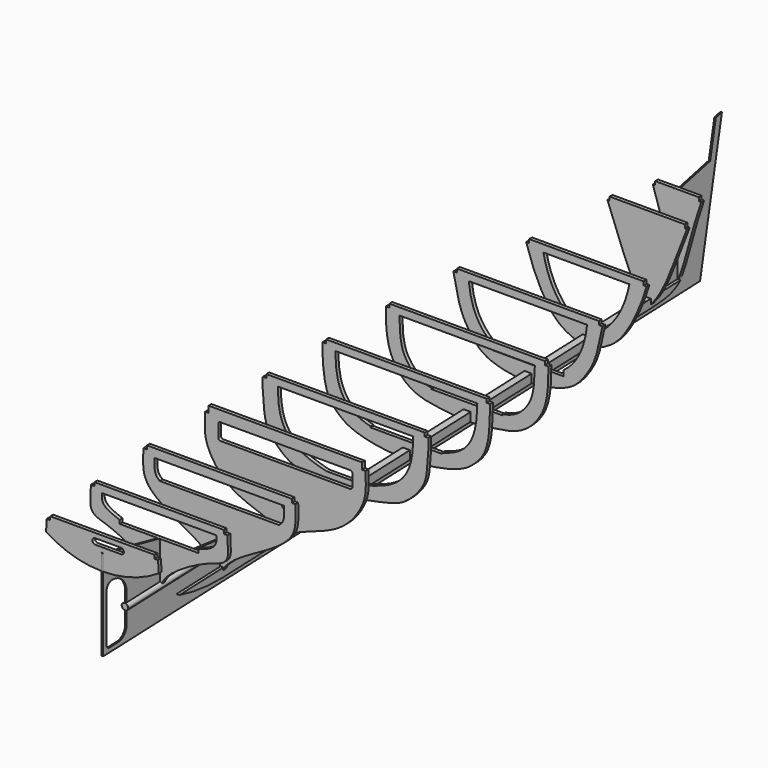
from build123d import *

# Parameters (mm, degrees)
F21_DEPTH      = 5
F11_W          = 160
F11_H          = 10
F22_DEPTH      = 5
F12_R          = 5
F12_W          = 181
F12_H          = 12
F23_DEPTH      = 5
F13_R          = 5
F24_DEPTH      = 5
F25_DEPTH      = 5
F15_W          = 114
F15_H          = 10
F26_DEPTH      = 5
F27_DEPTH      = 5
F28_DEPTH      = 5
F18_W          = 66
F18_H          = 10
F29_DEPTH      = 5
F30_DEPTH      = 5
F31_DEPTH      = 5
F33_DEPTH      = 1
F34_DEPTH      = 5
F36_R          = 4.4873534177
F37_DEPTH      = 2
F37_DEPTH_BACK = 170


# Not quite as in the source:
# - ends of sketch curves that miss each other by under 0.0002 mm in the source are joined
# - the dataset's text gives a spline's control points without its knots; the knots are read off the source's solid
# - a feature names something its author has since deleted; it is built from what else it names


with BuildPart() as f21:
    # F10 (on Front) → F21 (new body)
    with BuildSketch(Plane.XZ):
        with BuildLine():
            Line((72.7332957389, 50), (-72.7326870538, 50))
            Line((-72.7326870538, 50), (-72.7326870538, 45))
            Line((-72.7326870538, 45), (-77.7270149022, 45.2380952381))
            Line((-77.7270149022, 45.2380952381), (-78.5, 29.0238230366))
            ThreePointArc((-78.5, 29.0238230366), (-41.3829313198, 12.0162349326), (-1, 6.0034403622))
            Line((-1, 6.0034403622), (-1, 29.0034403622))
            Line((-1, 29.0034403622), (1, 29.0034403622))
            Line((1, 29.0034403622), (1, 6.0034403622))
            ThreePointArc((1, 6.0034403622), (41.3829313198, 12.0162349326), (78.5, 29.0238230366))
            Line((78.5, 29.0238230366), (77.7307292177, 45.1601830989))
            Line((77.7307292177, 45.1601830989), (72.7332957389, 45))
            Line((72.7332957389, 45), (72.7332957389, 50))
        make_face()
        with BuildLine():
            ThreePointArc((-10, 35.5), (-14, 39.5), (-10, 43.5))
            Line((-10, 43.5), (26, 43.5))
            ThreePointArc((26, 43.5), (30, 39.5), (26, 35.5))
            Line((26, 35.5), (-10, 35.5))
        make_face(mode=Mode.SUBTRACT)
    extrude(amount=-F21_DEPTH)


with BuildPart() as f22:
    # F11 (on offset) → F22 (new body)
    with BuildSketch(Plane.XZ.offset(-99)):
        with BuildLine():
            Line((-90.2041684767, 41), (-95.1998263135, 41.2083333333))
            Line((-95.1998263135, 41.2083333333), (-96, 22.0208423834))
            add(Edge.make_bspline(
                [(-96, 22.0208423834), (-96.9120721985, 5.4850967293), (-73.0751770721, 1.738031382), (-28.0955649636, -21.0631954445), (-7.6341264601, -38.9435383447), (-4, -48)],
                knots=[0, 0, 0, 0, 0.2926523272, 0.6814646887, 0.9688287938, 0.9688287938, 0.9688287938, 0.9688287938], degree=3))
            ThreePointArc((-4, -48), (-2.6742346142, -46.7752551286), (-1, -46.1010205144))
            Line((-1, -46.1010205144), (-1, -24.1010205144))
            Line((-1, -24.1010205144), (1, -24.1010205144))
            Line((1, -24.1010205144), (1, -46.1010205144))
            ThreePointArc((1, -46.1010205144), (2.6742346142, -46.7752551286), (4, -48))
            add(Edge.make_bspline(
                [(96, 22.0208423834), (96.9120721985, 5.4850967293), (73.0829633533, 1.7574750149), (28.0452981122, -21.1537837067), (7.6620989249, -38.8365497116), (4, -48)],
                knots=[0, 0, 0, 0, 0.2926523272, 0.6814646887, 0.969206891, 0.969206891, 0.969206891, 0.969206891], degree=3))
            Line((96, 22.0208423834), (95.2085144141, 41))
            Line((95.2085144141, 41), (90.2041684767, 41))
            Line((90.2041684767, 41), (90.2041684767, 46))
            Line((90.2041684767, 46), (80, 46))
            Line((80, 46), (80, 36))
            Line((80, 36), (80, 31))
            add(Edge.make_bspline(
                [(80, 31), (80, 18.6514444416), (67.1098306775, 14.6223076128), (55, 11.049054011)],
                knots=[0, 0, 0, 0, 31.985000326, 31.985000326, 31.985000326, 31.985000326], degree=3))
            Line((55, 11.049054011), (55, 6.049054011))
            Line((55, 6.049054011), (-55, 6.049054011))
            Line((-55, 6.049054011), (-55, 11.049054011))
            add(Edge.make_bspline(
                [(-80, 31), (-80, 18.6514444416), (-65.0256574154, 15.2740247987), (-55, 11.049054011)],
                knots=[0, 0, 0, 0, 31.985000326, 31.985000326, 31.985000326, 31.985000326], degree=3))
            Line((-80, 31), (-80, 36))
            Line((-80, 36), (-80, 46))
            Line((-80, 46), (-90.2041684767, 46))
            Line((-90.2041684767, 46), (-90.2041684767, 41))
        make_face()
        with Locations((0, 41)):
            Rectangle(F11_W, F11_H)
    extrude(amount=-F22_DEPTH)


with BuildPart() as f23:
    # F12 (on offset) → F23 (new body)
    with BuildSketch(Plane.XZ.offset(-204)):
        with BuildLine():
            Line((-90.5, 45), (-101, 45))
            Line((-101, 45), (-101, 40))
            Line((-101, 40), (-106, 40))
            add(Edge.make_bspline(
                [(-5, -74), (-8.813282499, -65.0429824265), (-34.1640834919, -44.0792117917), (-111.7253822581, -8.7611414274), (-106, 24.9656421202), (-106, 40)],
                knots=[0, 0, 0, 0, 0.2922002039, 0.7006643878, 1, 1, 1, 1], degree=3))
            Line((-5, -74), (-5, -70))
            Line((-5, -70), (5, -70))
            Line((5, -70), (5, -74))
            add(Edge.make_bspline(
                [(5, -74), (8.813282499, -65.0429824265), (34.1640834919, -44.0792117917), (111.7253822581, -8.7611414274), (106, 24.9656421202), (106, 40)],
                knots=[0, 0, 0, 0, 0.2922002039, 0.7006643878, 1, 1, 1, 1], degree=3))
            Line((106, 40), (101, 40))
            Line((101, 40), (101, 45))
            Line((101, 45), (90.5, 45))
            Line((90.5, 45), (90.5, 33))
            Line((90.5, 33), (90.5, 25))
            add(Edge.make_bspline(
                [(90.5, 25), (90.5, 13.7895681829), (87.9703567653, 10.8191042097), (83, 7)],
                knots=[0, 0, 0, 0, 19.5, 19.5, 19.5, 19.5], degree=3))
            Line((83, 7), (-83, 7))
            add(Edge.make_bspline(
                [(-90.5, 25), (-90.5, 13.7895681829), (-87.9703567653, 10.8191042097), (-83, 7)],
                knots=[0, 0, 0, 0, 19.5, 19.5, 19.5, 19.5], degree=3))
            Line((-90.5, 25), (-90.5, 33))
            Line((-90.5, 33), (-90.5, 45))
        make_face()
        with Locations((0, -46.9)):
            Circle(F12_R, mode=Mode.SUBTRACT)
        with Locations((0, 39)):
            Rectangle(F12_W, F12_H)
    extrude(amount=-F23_DEPTH)


with BuildPart() as f24:
    # F13 (on offset) → F24 (new body)
    with BuildSketch(Plane.XZ.offset(-319)):
        with BuildLine():
            add(Edge.make_bspline(
                [(112, 36), (112, 20.0375751766), (114.9710925703, 0.7454997503), (83.5609678216, -49.6149652842), (25.8806008493, -64.929650154), (11.6031311074, -72.9946899181), (5, -76.5)],
                knots=[0, 0, 0, 0, 0.2334395132, 0.5164907851, 0.8125057959, 1, 1, 1, 1], degree=3))
            Line((112, 36), (107, 36))
            Line((107, 36), (107, 45))
            Line((107, 45), (-107, 45))
            Line((-107, 45), (-107, 36))
            Line((-107, 36), (-112, 36))
            add(Edge.make_bspline(
                [(-112, 36), (-112, 20.0375751766), (-114.9710925703, 0.7454997503), (-83.5609678216, -49.6149652842), (-25.8806008493, -64.929650154), (-11.6031311074, -72.9946899181), (-5, -76.5)],
                knots=[0, 0, 0, 0, 0.2334395132, 0.5164907851, 0.8125057959, 1, 1, 1, 1], degree=3))
            Line((-5, -76.5), (-5, -66.5))
            Line((-5, -66.5), (5, -66.5))
            Line((5, -66.5), (5, -76.5))
        make_face()
        with Locations((0, -43)):
            Circle(F13_R, mode=Mode.SUBTRACT)
        with BuildLine():
            ThreePointArc((-93.5, 27), (-92.6213203436, 29.1213203436), (-90.5, 30))
            Line((-90.5, 30), (90.5, 30))
            ThreePointArc((90.5, 30), (92.6213203436, 29.1213203436), (93.5, 27))
            Line((93.5, 27), (93.5, 10))
            ThreePointArc((93.5, 10), (92.6213203436, 7.8786796564), (90.5, 7))
            Line((90.5, 7), (-90.5, 7))
            ThreePointArc((-90.5, 7), (-92.6213203436, 7.8786796564), (-93.5, 10))
            Line((-93.5, 10), (-93.5, 27))
        make_face(mode=Mode.SUBTRACT)
    extrude(amount=-F24_DEPTH)


with BuildPart() as f25:
    # F14 (on offset) → F25 (new body)
    with BuildSketch(Plane.XZ.offset(-424)):
        with BuildLine():
            add(Edge.make_bspline(
                [(-115.5, 20), (-115.3392433387, 13.9641281285), (-113.8140743497, -0.6317003896), (-112.0187554433, -26.2832826326), (-85.2145069128, -54.3299654785), (-62.9137435546, -63.2019640672), (-26.4105775656, -70.0387567849), (-5, -74)],
                knots=[0, 0, 0, 0, 0.1591894124, 0.3390317437, 0.5516980245, 0.7264384457, 1, 1, 1, 1], degree=3))
            Line((-5, -74), (-5, -62))
            Line((-5, -62), (5, -62))
            Line((5, -62), (5, -74))
            add(Edge.make_bspline(
                [(115.5, 20), (115.013504938, 13.502394231), (113.9868229516, -0.3893059037), (111.9517617805, -26.367587048), (85.2640044283, -54.3036345664), (62.7746395625, -63.2376778768), (26.8735338476, -69.9425419961), (5, -74)],
                knots=[0, 0, 0, 0, 0.1591894124, 0.3390317437, 0.5516980245, 0.7264384457, 1, 1, 1, 1], degree=3))
            Line((115.5, 20), (115.5, 35))
            Line((115.5, 35), (110.5, 35))
            Line((110.5, 35), (110.5, 40))
            Line((110.5, 40), (-110.5, 40))
            Line((-110.5, 40), (-110.5, 35))
            Line((-110.5, 35), (-115.5, 35))
            Line((-115.5, 35), (-115.5, 20))
        make_face()
        with BuildLine():
            Line((26.5, -52), (-26.5, -52))
            add(Edge.make_bspline(
                [(-94.5, 30), (-94.5409908891, -24.3969429284), (-74.9130025506, -39.9838760495), (-26.5, -52)],
                knots=[0, 0, 0, 0, 106.5269918847, 106.5269918847, 106.5269918847, 106.5269918847], degree=3))
            Line((-94.5, 30), (94.5, 30))
            add(Edge.make_bspline(
                [(94.5, 30), (94.5409908891, -24.3969429284), (74.9130025506, -39.9838760495), (26.5, -52)],
                knots=[0, 0, 0, 0, 106.5269918847, 106.5269918847, 106.5269918847, 106.5269918847], degree=3))
        make_face(mode=Mode.SUBTRACT)
    extrude(amount=-F25_DEPTH)


with BuildPart() as f26:
    # F15 (on offset) → F26 (new body)
    with BuildSketch(Plane.XZ.offset(-530)):
        with BuildLine():
            Line((57, 29), (99, 29))
            add(Edge.make_bspline(
                [(99, 29), (98.8524481654, -23.819649592), (81.244982779, -39.1179360449), (50, -47.5)],
                knots=[0, 0, 0, 0, 90.8473995225, 90.8473995225, 90.8473995225, 90.8473995225], degree=3))
            Line((50, -47.5), (50, -49))
            Line((50, -49), (-50, -49))
            Line((-50, -49), (-50, -47.5))
            add(Edge.make_bspline(
                [(-99, 29), (-98.8524481654, -23.819649592), (-81.244982779, -39.1179360449), (-50, -47.5)],
                knots=[0, 0, 0, 0, 90.8473995225, 90.8473995225, 90.8473995225, 90.8473995225], degree=3))
            Line((-99, 29), (-57, 29))
            Line((-57, 29), (-57, 39))
            Line((-57, 39), (-112, 39))
            Line((-112, 39), (-112, 34))
            Line((-112, 34), (-117, 34))
            add(Edge.make_bspline(
                [(-117, 34), (-117.1332637698, 16.7322402547), (-116.2505094659, 2.9696295502), (-110.9819940422, -31.2896778126), (-91.9333809233, -49.8180802014), (-74.7177469914, -61.4927914834), (-35.4341869017, -71.341135338), (-5, -71)],
                knots=[0, 0, 0, 0, 0.199598267, 0.3898589499, 0.5603797965, 0.71066453, 1, 1, 1, 1], degree=3))
            Line((-5, -71), (-5, -59))
            Line((-5, -59), (5, -59))
            Line((5, -59), (5, -71))
            add(Edge.make_bspline(
                [(117, 34), (116.8018199388, 22.6155687523), (116.3975171997, 0.3601533472), (110.9477316202, -30.6814990963), (91.940843165, -49.9505395061), (74.713668487, -61.420395564), (35.4341869017, -71.341135338), (5, -71)],
                knots=[0, 0, 0, 0, 0.199598267, 0.3898589499, 0.5603797965, 0.71066453, 1, 1, 1, 1], degree=3))
            Line((117, 34), (112, 34))
            Line((112, 34), (112, 39))
            Line((112, 39), (57, 39))
            Line((57, 39), (57, 29))
        make_face()
        with Locations((0, 34)):
            Rectangle(F15_W, F15_H)
    extrude(amount=-F26_DEPTH)


with BuildPart() as f27:
    # F16 (on offset) → F27 (new body)
    with BuildSketch(Plane.XZ.offset(-636)):
        with BuildLine():
            Line((108.5, 41), (-108.5, 41))
            Line((-108.5, 41), (-108.5, 36))
            Line((-108.5, 36), (-113.5, 36))
            add(Edge.make_bspline(
                [(-113.5, 36), (-113.6853100213, 23.2057292639), (-112.6767038788, 0.3110175039), (-105.7737152566, -25.2638223347), (-89.8461490834, -45.8472691617), (-69.1078103598, -59.7110377935), (-48.5849191801, -64.1945032488), (-5, -68)],
                knots=[0, 0, 0, 0, 0.2082797969, 0.3854896789, 0.5589225093, 0.7117658935, 1, 1, 1, 1], degree=3))
            Line((-5, -68), (-5, -56))
            Line((-5, -56), (5, -56))
            Line((5, -56), (5, -68))
            add(Edge.make_bspline(
                [(113.5, 36), (113.6853100213, 23.2057292639), (112.6767038788, 0.3110175039), (105.7737152566, -25.2638223347), (89.8461490834, -45.8472691617), (69.1078103598, -59.7110377935), (48.5849191801, -64.1945032488), (5, -68)],
                knots=[0, 0, 0, 0, 0.2082797969, 0.3854896789, 0.5589225093, 0.7117658935, 1, 1, 1, 1], degree=3))
            Line((113.5, 36), (108.5, 36))
            Line((108.5, 36), (108.5, 41))
        make_face()
        with BuildLine():
            Line((49.5, -45), (-49.5, -45))
            Line((-49.5, -45), (-49.5, -43.5))
            add(Edge.make_bspline(
                [(-94.4999861866, 31.0000001116), (-94.497941227, 28.9956921132), (-94.4345897257, 23.4907172125), (-94.1261702571, 16.5300619118), (-93.6028668535, 10.1839720209), (-93.0972465835, 5.6618996543), (-92.4785534037, 1.4027750015), (-91.7559378079, -2.5042294246), (-90.9164595905, -6.0906713906), (-89.9489761016, -9.3969663235), (-89.0227202168, -11.9646425883), (-88.1973581885, -13.9386492915), (-87.5308292824, -15.3898018715), (-86.8151567539, -16.8137333348), (-86.0251311751, -18.2574076758), (-85.1665936431, -19.7093942543), (-83.9394412981, -21.6416479823), (-82.2685633433, -24.0234959768), (-80.1081545618, -26.7481277375), (-77.8628105033, -29.2658031409), (-75.6191047077, -31.4992174217), (-73.45542822, -33.396976559), (-71.3076445092, -35.0442343421), (-69.4753331717, -36.2646697204), (-67.9442871638, -37.1797447189), (-66.7526930847, -37.8416160147), (-65.511068482, -38.4827897218), (-64.1990830505, -39.113073092), (-62.9040334978, -39.6891753625), (-61.1198452723, -40.415567772), (-58.6577772593, -41.2834732934), (-54.9482494439, -42.3332813547), (-51.6364309743, -43.0778677009), (-49.6605637637, -43.468553636), (-49.5, -43.5)],
                knots=[0.0273700449, 0.0273700449, 0.0273700449, 0.0273700449, 0.0625, 0.125, 0.15625, 0.1875, 0.21875, 0.25, 0.28125, 0.3125, 0.34375, 0.359375, 0.375, 0.390625, 0.40625, 0.421875, 0.4375, 0.46875, 0.5, 0.53125, 0.5625, 0.59375, 0.625, 0.65625, 0.671875, 0.6875, 0.703125, 0.71875, 0.734375, 0.75, 0.78125, 0.8125, 0.84375, 0.8464833531, 0.8464833531, 0.8464833531, 0.8464833531], degree=3))
            Line((-94.4999861866, 31.0000001116), (94.5, 31))
            add(Edge.make_bspline(
                [(94.5, 31), (94.497941227, 28.9956921132), (94.4345897257, 23.4907172125), (94.1261702571, 16.5300619118), (93.6028668535, 10.1839720209), (93.0972465835, 5.6618996544), (92.4785534037, 1.4027750016), (91.7559378079, -2.5042294246), (90.9164595905, -6.0906713906), (89.9489761016, -9.3969663235), (89.0227202167, -11.9646425883), (88.1973581885, -13.9386492916), (87.5308292823, -15.3898018716), (86.8151567539, -16.8137333349), (86.0251311751, -18.2574076759), (85.166593643, -19.7093942544), (83.9394412981, -21.6416479824), (82.2685633433, -24.0234959768), (80.1081545619, -26.7481277375), (77.8628105035, -29.2658031408), (75.619104708, -31.4992174214), (73.4554282202, -33.3969765587), (71.3076445091, -35.044234342), (69.4753331715, -36.2646697204), (67.9442871634, -37.179744719), (66.7526930841, -37.8416160149), (65.5110684814, -38.4827897221), (64.1990830498, -39.1130730924), (62.9040334972, -39.6891753629), (61.119845272, -40.4155677724), (58.6577772596, -41.2834732936), (54.9482494451, -42.3332813549), (51.6364309761, -43.077867701), (49.6605637657, -43.4685536361), (49.4999989755, -43.4999950591)],
                knots=[0.0273700449, 0.0273700449, 0.0273700449, 0.0273700449, 0.0625, 0.125, 0.15625, 0.1875, 0.21875, 0.25, 0.28125, 0.3125, 0.34375, 0.359375, 0.375, 0.390625, 0.40625, 0.421875, 0.4375, 0.46875, 0.5, 0.53125, 0.5625, 0.59375, 0.625, 0.65625, 0.671875, 0.6875, 0.703125, 0.71875, 0.734375, 0.75, 0.78125, 0.8125, 0.84375, 0.8464833531, 0.8464833531, 0.8464833531, 0.8464833531], degree=3))
            Line((49.4999989755, -43.4999950591), (49.5, -45))
        make_face(mode=Mode.SUBTRACT)
    extrude(amount=-F27_DEPTH)


with BuildPart() as f28:
    # F17 (on offset) → F28 (new body)
    with BuildSketch(Plane.XZ.offset(-742)):
        with BuildLine():
            Line((99, 44), (-99, 44))
            Line((-99, 44), (-99, 39))
            Line((-99, 39), (-104, 39))
            add(Edge.make_bspline(
                [(-104, 39), (-101.3474084727, 27.10401983), (-96.8988978989, -0.4246595204), (-83.8941602942, -24.689924803), (-71.8735231329, -40.5831131104), (-55.8881544858, -53.9052198311), (-29.9967527393, -60.9264485588), (-5, -63)],
                knots=[0, 0, 0, 0, 0.2299594934, 0.4213706733, 0.579396756, 0.7344656492, 1, 1, 1, 1], degree=3))
            Line((-5, -63), (-5, -51))
            Line((-5, -51), (5, -51))
            Line((5, -51), (5, -63))
            add(Edge.make_bspline(
                [(104, 39), (101.3474084727, 27.10401983), (96.8988978989, -0.4246595204), (83.8941602942, -24.689924803), (71.8735231329, -40.5831131104), (55.8881544858, -53.9052198311), (29.9967527393, -60.9264485588), (5, -63)],
                knots=[0, 0, 0, 0, 0.2299594934, 0.4213706733, 0.579396756, 0.7344656492, 1, 1, 1, 1], degree=3))
            Line((104, 39), (99, 39))
            Line((99, 39), (99, 44))
        make_face()
        with BuildLine():
            add(Edge.make_bspline(
                [(-82.5, 34), (-79.4951915741, 5.5740713142), (-70.7563683391, -16.2057764828), (-50, -32)],
                knots=[0, 0, 0, 0, 73.567995759, 73.567995759, 73.567995759, 73.567995759], degree=3))
            Line((-82.5, 34), (82.5, 34))
            add(Edge.make_bspline(
                [(50, -32), (70.7563683391, -16.2057764828), (79.4951915741, 5.5740713142), (82.5, 34)],
                knots=[0, 0, 0, 0, 73.567995759, 73.567995759, 73.567995759, 73.567995759], degree=3))
            Line((50, -32), (50, -40))
            Line((50, -40), (-50, -40))
            Line((-50, -40), (-50, -32))
        make_face(mode=Mode.SUBTRACT)
    extrude(amount=-F28_DEPTH)


with BuildPart() as f29:
    # F18 (on offset) → F29 (new body)
    with BuildSketch(Plane.XZ.offset(-844)):
        with BuildLine():
            Line((-33, 45), (-80, 45))
            Line((-80, 45), (-80, 40))
            Line((-80, 40), (-84, 40))
            add(Edge.make_bspline(
                [(-84, 40), (-79.8447122589, 26.2744808848), (-70.3764042593, 0.2208752669), (-52.1780151891, -31.5230981427), (-34.2026744377, -49.8146207054), (-14.985605143, -58.1584945321), (-5, -60.5)],
                knots=[0, 0, 0, 0, 0.2835218964, 0.5432366791, 0.7605814027, 1, 1, 1, 1], degree=3))
            Line((-5, -60.5), (-5, -48.5))
            Line((-5, -48.5), (5, -48.5))
            Line((5, -48.5), (5, -60.5))
            add(Edge.make_bspline(
                [(5, -60.5), (14.985605143, -58.1584945321), (34.2026744377, -49.8146207054), (52.1780151891, -31.5230981427), (70.3764042593, 0.2208752669), (79.8447122589, 26.2744808848), (84, 40)],
                knots=[0, 0, 0, 0, 0.2394185973, 0.4567633209, 0.7164781036, 1, 1, 1, 1], degree=3))
            Line((84, 40), (80, 40))
            Line((80, 40), (80, 45))
            Line((80, 45), (33, 45))
            Line((33, 45), (33, 35))
            Line((33, 35), (60, 35))
            add(Edge.make_bspline(
                [(60, 35), (54.4112771749, 9.017445147), (45.7816235721, -11.9644580409), (26, -31)],
                knots=[0, 0, 0, 0, 74.2428447731, 74.2428447731, 74.2428447731, 74.2428447731], degree=3))
            Line((26, -31), (-26, -31))
            add(Edge.make_bspline(
                [(-60, 35), (-54.4112771749, 9.017445147), (-45.7816235721, -11.9644580409), (-26, -31)],
                knots=[0, 0, 0, 0, 74.2428447731, 74.2428447731, 74.2428447731, 74.2428447731], degree=3))
            Line((-60, 35), (-33, 35))
            Line((-33, 35), (-33, 45))
        make_face()
        with Locations((0, 40)):
            Rectangle(F18_W, F18_H)
    extrude(amount=-F29_DEPTH)


with BuildPart() as f30:
    # F19 (on offset) → F30 (new body)
    with BuildSketch(Plane.XZ.offset(-950)):
        with BuildLine():
            Line((52.5, 63), (-52.5, 63))
            Line((-52.5, 63), (-52.5, 58))
            Line((-52.5, 58), (-55.4554026298, 58))
            add(Edge.make_bspline(
                [(-55.4554026298, 58), (-47.4490426725, 38.2374866556), (-33.0784365178, -1.4228418433), (-18.2192102075, -35.8350165188), (-5, -51)],
                knots=[0.0403525547, 0.0403525547, 0.0403525547, 0.0403525547, 0.5187409145, 1, 1, 1, 1], degree=3))
            Line((-5, -51), (-5, -44))
            Line((-5, -44), (5, -44))
            Line((5, -44), (5, -51))
            add(Edge.make_bspline(
                [(5, -51), (18.2192102075, -35.8350165188), (33.0784365178, -1.4228418433), (47.4490426725, 38.2374866556), (55.4554026298, 58)],
                knots=[0, 0, 0, 0, 0.4812590855, 0.9596474453, 0.9596474453, 0.9596474453, 0.9596474453], degree=3))
            Line((55.4554026298, 58), (52.5, 58))
            Line((52.5, 58), (52.5, 63))
        make_face()
    extrude(amount=-F30_DEPTH)


with BuildPart() as f31:
    # F20 (on offset) → F31 (new body)
    with BuildSketch(Plane.XZ.offset(-1002)):
        with BuildLine():
            Line((30.5, 68), (-30.5, 68))
            Line((-30.5, 68), (-30.5, 63))
            Line((-30.5, 63), (-33.767692073, 63))
            add(Edge.make_bspline(
                [(-33.767692073, 63), (-24.5677720814, 36.1729161403), (-15.7664325554, 2.2370271), (-7.0536155688, -28.9400164466), (-2, -42)],
                knots=[0.0321525257, 0.0321525257, 0.0321525257, 0.0321525257, 0.5596628697, 1, 1, 1, 1], degree=3))
            Line((-2, -42), (-1, -42))
            Line((-1, -42), (-1, 20))
            Line((-1, 20), (1, 20))
            Line((1, 20), (1, -42))
            Line((1, -42), (2, -42))
            add(Edge.make_bspline(
                [(2, -42), (7.0536155688, -28.9400164466), (15.7664325554, 2.2370271), (24.5677720814, 36.1729161403), (33.767692073, 63)],
                knots=[0, 0, 0, 0, 0.4403371303, 0.9678474743, 0.9678474743, 0.9678474743, 0.9678474743], degree=3))
            Line((33.767692073, 63), (30.5, 63))
            Line((30.5, 63), (30.5, 68))
        make_face()
    extrude(amount=-F31_DEPTH)


with BuildPart() as f33:
    # F32 (on Right) → F33 (new body, symmetric)
    with BuildSketch(Plane.YZ):
        with BuildLine():
            Line((204, -70.7867812279), (203.8923381653, -52.7787993088))
            Line((203.8923381653, -52.7787993088), (41, -58.7021570603))
            Line((41, -58.7021570603), (41, -76.258847562))
            ThreePointArc((41, -76.258847562), (36.7976019114, -86.6709459559), (26.5450942716, -91.2489400312))
            Line((26.5450942716, -91.2489400312), (11.1816980905, -91.8076089833))
            ThreePointArc((11.1816980905, -91.8076089833), (7.5293005354, -90.4101121307), (6, -86.8109114935))
            Line((6, -86.8109114935), (6, -20.5812143789))
            ThreePointArc((6, -20.5812143789), (8.9036014217, -13.5355684031), (15.9282254435, -10.5814719616))
            ThreePointArc((15.9282254435, -10.5814719616), (33.7217767745, -17.8398315591), (41.1076618347, -35.5808280049))
            Line((41.1076618347, -35.5808280049), (41.1076618347, -48.6916326984))
            Line((41.1076618347, -48.6916326984), (204, -42.768274947))
            Line((204, -42.768274947), (204, -36.768274947))
            Line((204, -36.768274947), (99, -24.5719161158))
            Line((99, -24.5719161158), (99, 6.4485729809))
            Line((99, 6.4485729809), (0, 28))
            Line((0, 28), (0, -98))
            Line((0, -98), (6, -98))
            Line((6, -98), (204, -90.8))
            Line((204, -90.8), (204, -82.7947124912))
            add(Edge.make_bspline(
                [(128, -73.5504175915), (152.1387539332, -80.1153257797), (177.6528805492, -83.5033804179), (204, -82.7947124912)],
                knots=[0, 0, 0, 0, 76.560152744, 76.560152744, 76.560152744, 76.560152744], degree=3))
            Line((128, -73.5504175915), (204, -70.7867812279))
        make_face()
        with BuildLine():
            Line((204, -82.7947124912), (204, -70.7867812279))
            Line((204, -70.7867812279), (128, -73.5504175915))
            add(Edge.make_bspline(
                [(128, -73.5504175915), (152.1387539332, -80.1153257797), (177.6528805492, -83.5033804179), (204, -82.7947124912)],
                knots=[0, 0, 0, 0, 76.560152744, 76.560152744, 76.560152744, 76.560152744], degree=3))
        make_face()
        Polygon((955, -43.4776903188), (204, -70.7867812279), (204, -82.7947124912), (955, -55.4856215821), align=None)
        Polygon((955, -55.4856215821), (204, -82.7947124912), (204, -90.8), (955, -63.4909090909), align=None)
        with BuildLine():
            Line((955, -6.4776903188), (955, -43.4776903188))
            Line((955, -43.4776903188), (1001.9689564035, -41.7697282678))
            add(Edge.make_bspline(
                [(955, -55.4856215821), (971.896469593, -54.6807125211), (989.3863797188, -53.2584600151), (1001.9689564035, -41.7697282678)],
                knots=[0, 0, 0, 0, 48.9306508749, 48.9306508749, 48.9306508749, 48.9306508749], degree=3))
            Line((955, -55.4856215821), (955, -63.4909090909))
            Line((955, -63.4909090909), (1040.9431968234, -60.3657019337))
            Line((1040.9431968234, -60.3657019337), (1079.0518338969, 131.5268630311))
            Line((1079.0518338969, 131.5268630311), (1068.3631160052, 129.0422528858))
            Line((1068.3631160052, 129.0422528858), (1058.6236379966, 80))
            Line((1058.6236379966, 80), (1007, 68))
            Line((1007, 68), (1007, 19))
            Line((1007, 19), (1002, 19))
            Line((1002, 19), (955, -6.4776903188))
        make_face()
        with BuildLine():
            Line((1001.9689564035, -41.7697282678), (955, -43.4776903188))
            Line((955, -43.4776903188), (955, -55.4856215821))
            add(Edge.make_bspline(
                [(955, -55.4856215821), (971.896469593, -54.6807125211), (989.3863797188, -53.2584600151), (1001.9689564035, -41.7697282678)],
                knots=[0, 0, 0, 0, 48.9306508749, 48.9306508749, 48.9306508749, 48.9306508749], degree=3))
        make_face()
    extrude(amount=F33_DEPTH, both=True)

    # F32 (on Right) → F34 (join, symmetric)
    with BuildSketch(Plane.YZ):
        with BuildLine():
            Line((204, -82.7947124912), (204, -70.7867812279))
            Line((204, -70.7867812279), (128, -73.5504175915))
            add(Edge.make_bspline(
                [(128, -73.5504175915), (152.1387539332, -80.1153257797), (177.6528805492, -83.5033804179), (204, -82.7947124912)],
                knots=[0, 0, 0, 0, 76.560152744, 76.560152744, 76.560152744, 76.560152744], degree=3))
        make_face()
        Polygon((955, -43.4776903188), (204, -70.7867812279), (204, -82.7947124912), (955, -55.4856215821), align=None)
        with BuildLine():
            Line((1001.9689564035, -41.7697282678), (955, -43.4776903188))
            Line((955, -43.4776903188), (955, -55.4856215821))
            add(Edge.make_bspline(
                [(955, -55.4856215821), (971.896469593, -54.6807125211), (989.3863797188, -53.2584600151), (1001.9689564035, -41.7697282678)],
                knots=[0, 0, 0, 0, 48.9306508749, 48.9306508749, 48.9306508749, 48.9306508749], degree=3))
        make_face()
    extrude(amount=F34_DEPTH, both=True)


with BuildPart() as f37:
    # F36 (on line) → F37 (new body, two sides)
    with BuildSketch(Plane(origin=(0, 39.2851097568, 1.4285494457), x_dir=(1, 0, 0), z_dir=(0, -0.9993394979, -0.0363396181))) as f37_sk:
        with Locations((0, -54.6406619251)):
            Circle(F36_R)
    extrude(amount=F37_DEPTH)
    extrude(f37_sk.sketch, amount=-F37_DEPTH_BACK)


solid = Compound([f21.part, f22.part, f23.part, f24.part, f25.part, f26.part, f27.part, f28.part, f29.part, f30.part, f31.part, f33.part, f37.part])
